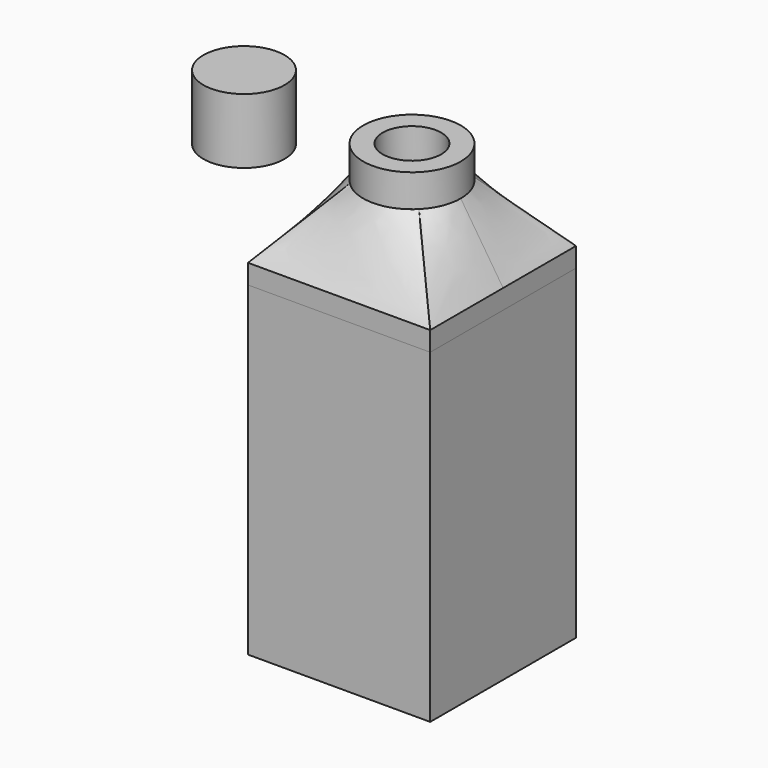
from build123d import *

# Parameters (mm, degrees)
F0_W      = 28
F0_H      = 28
F0_W_2    = 22
F0_H_2    = 22
F1_DEPTH  = 50
F2_DEPTH  = 20
F3_W      = 28
F3_H      = 28
F3_W_2    = 22
F3_H_2    = 22
F4_DEPTH  = 3
F5_R      = 6.2368420166
F6_DEPTH  = 10
F7_R      = 7.5
F8_DEPTH  = 5
F8_FACE_R = 7.5
F4_FACE_W = 28
F4_FACE_H = 28
F10_R     = 4.5
F11_DEPTH = 200


with BuildPart() as f1:
    # F0 (on Top) → F1 (new body)
    with BuildSketch(Plane.XY):
        with Locations((-21.8676342088, 13.622631086)):
            Rectangle(F0_W, F0_H)
        with Locations((-21.8676342088, 13.622631086)):
            Rectangle(F0_W_2, F0_H_2, mode=Mode.SUBTRACT)
    extrude(amount=F1_DEPTH)

    # F0 (on Top) → F2 (join)
    with BuildSketch(Plane.XY):
        with Locations((-21.8676342088, 13.622631086)):
            Rectangle(F0_W_2, F0_H_2)
    extrude(amount=F2_DEPTH)


with BuildPart() as f4:
    # F3 (on face) → F4 (new body)
    with BuildSketch(Plane.XY.offset(50)):
        with Locations((-21.8676342088, 13.622631086)):
            Rectangle(F3_W, F3_H)
        with Locations((-21.8676342088, 13.622631086)):
            Rectangle(F3_W_2, F3_H_2, mode=Mode.SUBTRACT)
        with Locations((-21.8676342088, 13.622631086)):
            Rectangle(F3_W_2, F3_H_2)
    extrude(amount=F4_DEPTH)

    # F8_face (on face) → F9 section 0
    with BuildSketch(Plane(origin=(-21.8676342088, 13.622631086, 63), x_dir=(1, 0, 0), z_dir=(0, 0, -1))):
        Circle(F8_FACE_R)
    # F4_face (on face) → F9 section 1
    with BuildSketch(Plane(origin=(-21.8676342088, 13.622631086, 53), x_dir=(1, 0, 0), z_dir=(0, 0, 1))):
        Rectangle(F4_FACE_W, F4_FACE_H)
    loft()


with BuildPart() as f6:
    # F5 (on face) → F6 (new body)
    with BuildSketch(Plane.XY.offset(53)):
        with Locations((-55.5168837309, 23.41972664)):
            Circle(F5_R)
    extrude(amount=F6_DEPTH)


with BuildPart() as f8:
    # F7 (on face) → F8 (new body)
    with BuildSketch(Plane.XY.offset(63)):
        with Locations((-21.8676342088, 13.622631086)):
            Circle(F7_R)
    extrude(amount=F8_DEPTH)

    # F10 (on face) + F7 (on face) + F5 (on face) → F11 (cut)
    with BuildSketch(Plane.XY.offset(68)):
        with Locations((-21.8676342088, 13.622631086)):
            Circle(F10_R)
    with BuildSketch(Plane.XY.offset(63)):
        with Locations((-21.8676342088, 13.622631086)):
            Circle(F7_R)
    with BuildSketch(Plane.XY.offset(53)):
        with Locations((-55.5168837309, 23.41972664)):
            Circle(F5_R)
    extrude(amount=-F11_DEPTH, mode=Mode.SUBTRACT)


solid = Compound([f1.part, f4.part, f6.part, f8.part])
